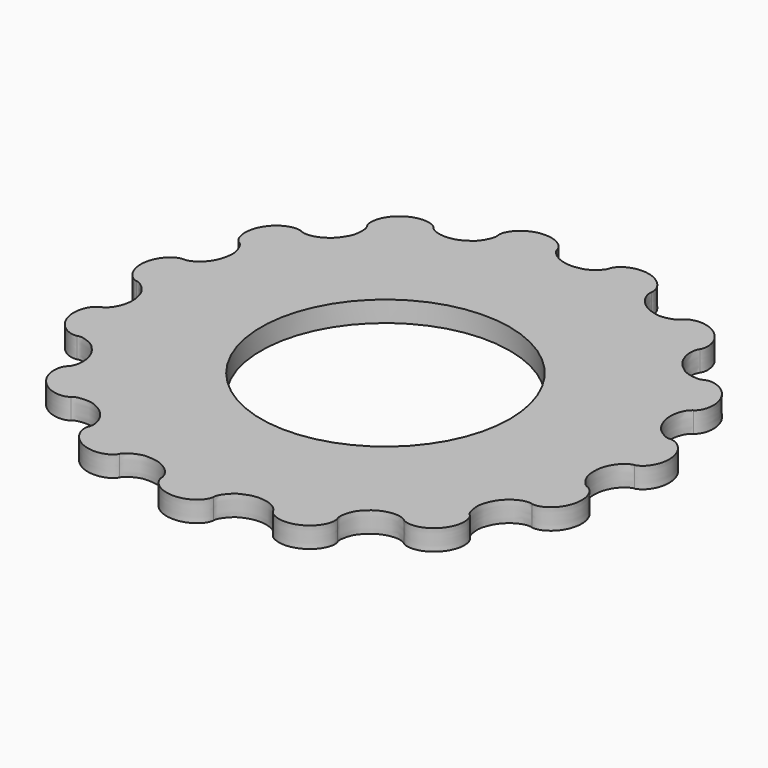
from build123d import *

# Parameters (mm, degrees)
F1_R            = 30
F2_DEPTH        = 2.5
F4_DEPTH        = 2.5
F4_COPIES_COUNT = 15
F6_DEPTH        = 2.5010001
F6_COPIES_COUNT = 15
F7_R            = 15
F8_DEPTH        = 2.5010001


# Not quite as in the source:
# - a pattern or mirror of a feature is missing from the dataset's text; its kind, count and spacing are read off the source's solid


with BuildPart() as f2:
    # F1 (on Top) → F2 (new body)
    with BuildSketch(Plane.XY):
        Circle(F1_R)
    extrude(amount=F2_DEPTH)

    # F3 (on face) → F4 (join, through all)
    with BuildSketch(Plane.XY.offset(2.5)):
        with BuildLine():
            add(Edge.make_bspline(
                [(29.344428022, 6.2373507245), (29.3933354021, 6.2477463091), (29.4907818104, 6.2458927428), (29.9260713153, 6.1668744849), (30.4933926149, 5.8549659014), (31.1158428866, 5.2590115229), (31.614702741, 4.3921350903), (31.874991761, 3.3501963002), (31.8370218419, 2.2769099498), (31.5292969648, 1.3252579493), (31.0443549487, 0.6129120372), (30.5542793765, 0.189866424), (30.1449362259, 0.0220748714), (30.049999975, 0), (30, 4.9956e-05)],
                knots=[0, 0, 0, 0, 0.0392231241, 0.1063510743, 0.1910134394, 0.2876620616, 0.3919582226, 0.5000006598, 0.6080430653, 0.7123392263, 0.8089878485, 0.8936502136, 0.9607781638, 1, 1, 1, 1], degree=3))
            ThreePointArc((29.344428022, 6.2373507245), (29.3977411386, 5.9810380325), (29.4488155034, 5.7242698613))
            ThreePointArc((29.4488155034, 5.7242698613), (29.4976472269, 5.4670657648), (29.5442325904, 5.20944533))
            ThreePointArc((29.5442325904, 5.20944533), (29.8858387658, 2.6146971654), (30, 4.9956e-05))
        make_face()
        with BuildLine():
            add(Edge.make_bspline(
                [(2.5968880159, 2.4969243124), (2.6457953959, 2.507319897), (2.7432418043, 2.5054663307), (3.1785313092, 2.4264480726), (3.7458526087, 2.1145394897), (4.3683028807, 1.5185851084), (4.8671627373, 0.6517086817), (5.1274517595, -0.390230156), (5.0894818326, -1.4635164595), (4.7817569589, -2.4151684652), (4.2968149425, -3.1275143744), (3.8067393704, -3.5505599883), (3.3973962198, -3.7183515408), (3.3024599689, -3.7404264122), (3.2524599938, -3.7403764563)],
                knots=[0, 0, 0, 0, 0.0392231241, 0.1063510743, 0.1910134394, 0.2876620616, 0.3919582226, 0.5000006619, 0.6080430653, 0.7123392263, 0.8089878485, 0.8936502136, 0.9607781638, 1, 1, 1, 1], degree=3))
            ThreePointArc((2.5968880159, 2.4969243124), (2.6502011325, 2.2406116204), (2.7012754973, 1.9838434492))
            ThreePointArc((2.7012754973, 1.9838434492), (2.7501072208, 1.7266393526), (2.7966925842, 1.4690189179))
            ThreePointArc((2.7966925842, 1.4690189179), (3.1382987596, -1.1257292468), (3.2524599938, -3.7403764563))
        make_face()
    f4 = extrude(amount=-F4_DEPTH)

    # F4_copies: F4 ×15 about axis
    f4_copies_axis = Axis((0, 0, 0), (0, 0, 1))
    for i in range(1, F4_COPIES_COUNT):
        add(f4.rotate(f4_copies_axis, i * 360 / F4_COPIES_COUNT))

    # F5 (on face) → F6 (cut, through all)
    with BuildSketch(Plane.XY.offset(2.5)):
        with BuildLine():
            ThreePointArc((27.6151456036, 11.7219338547), (27.5118022316, 11.9624720678), (27.4063637293, 12.2020992923))
            add(Edge.make_bspline(
                [(29.344428022, 6.2373507245), (29.295520642, 6.22695514), (29.2022743002, 6.233123582), (28.7746198394, 6.2419232171), (27.5472761579, 6.9892563869), (27.043052587, 7.71669433), (26.5824231035, 8.6436931859), (26.4014788587, 9.6227803042), (26.4464444164, 10.5561239597), (26.685775911, 11.3246501923), (26.9886897968, 11.8453432179), (27.2921046088, 12.1314608661), (27.3606864564, 12.1817624601), (27.4063637293, 12.2020992923)],
                knots=[0, 0, 0, 0, 0.0414260396, 0.1123321793, 0.2475649801, 0.3577326485, 0.4718575381, 0.5859823857, 0.6961500541, 0.7982395608, 0.8876678207, 0.9585739604, 1, 1, 1, 1], degree=3))
            ThreePointArc((29.344428022, 6.2373507245), (28.6115085224, 9.0211739851), (27.6151456036, 11.7219338547))
        make_face()
    f6 = extrude(amount=-F6_DEPTH, mode=Mode.SUBTRACT)

    # F6_copies: F6 ×15 about axis
    f6_copies_axis = Axis((0, 0, 0), (0, 0, 1))
    for i in range(1, F6_COPIES_COUNT):
        add(f6.rotate(f6_copies_axis, i * 360 / F6_COPIES_COUNT), mode=Mode.SUBTRACT)

    # F7 (on face) → F8 (cut, through all)
    with BuildSketch(Plane.XY.offset(2.5)):
        Circle(F7_R)
    extrude(amount=-F8_DEPTH, mode=Mode.SUBTRACT)


solid = f2.part
